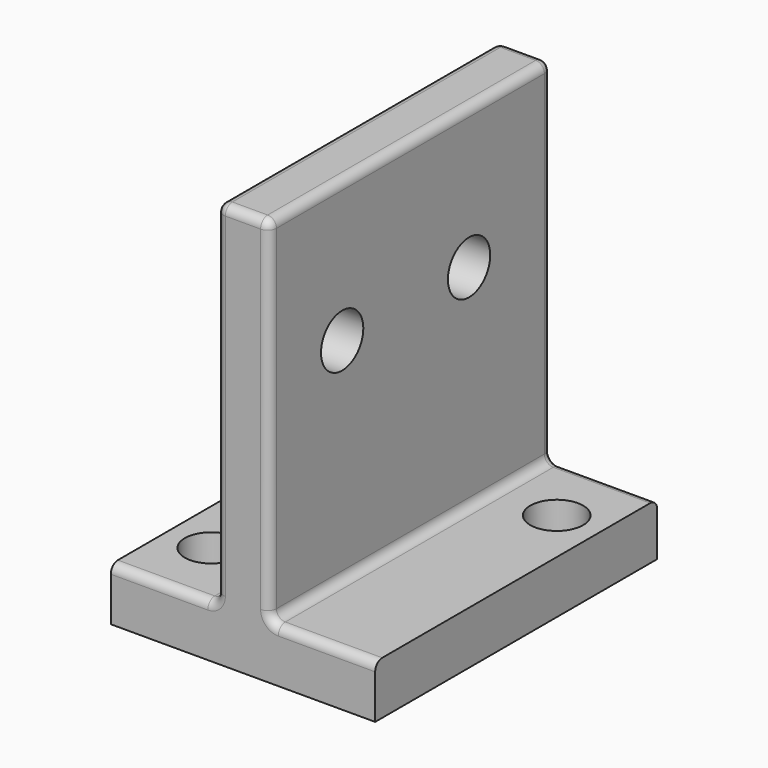
from build123d import *

# Parameters (mm, degrees)
F0_W     = 3
F0_H     = 20
F1_DEPTH = 20
F2_R     = 1.5
F3_DEPTH = 9.001
F4_R     = 1.5
F5_DEPTH = 3.001
F6_R     = 1.5
F7_DEPTH = 25
F8_F1_R  = 0.5
F8_F2_R  = 0.5


with BuildPart() as f1:
    # F0 (on Front) → F1 (new body)
    with BuildSketch(Plane.XZ):
        Rectangle(F0_W, F0_H)
        Polygon((7.5, -10), (1.5, -10), (-1.5, -10), (-7.5, -10), (-7.5, -13), (7.5, -13), align=None)
    extrude(amount=F1_DEPTH)

    # F2 (on face) → F3 (cut, through all)
    with BuildSketch(Plane.YZ.offset(1.5)):
        with Locations((-14.8428049088, 2)):
            Circle(F2_R)
        with Locations((-5.8428049088, 2)):
            Circle(F2_R)
    extrude(amount=-F3_DEPTH, mode=Mode.SUBTRACT)

    # F4 (on face) → F5 (cut, through all)
    with BuildSketch(Plane.XY.offset(-10)):
        with Locations((5, -4)):
            Circle(F4_R)
    extrude(amount=-F5_DEPTH, mode=Mode.SUBTRACT)

    # F6 (on face) → F7 (cut)
    with BuildSketch(Plane.XY.offset(-10)):
        with Locations((-5, -16)):
            Circle(F6_R)
    extrude(amount=-F7_DEPTH, mode=Mode.SUBTRACT)

    # F8: fillet of radius 0.5 on 10 edges, made by hand

    # F8_f1
    f8_f1_edges = [f1.edges().sort_by_distance(p)[0] for p in [
        (1.5, -10, -10),
        (-1.5, -10, -10),
    ]]
    fillet(f8_f1_edges, radius=F8_F1_R)

    # F8_f2
    f8_f2_edges = [f1.edges().sort_by_distance(p)[0] for p in [
        (-1.5, -10, 10),
        (1.5, -20, 0.25),
        (-1.5, -20, 0.25),
        (1.5, -10, 10),
        (-1.5, 0, 0.25),
        (1.5, 0, 0.25),
        (0, -20, 10),
        (0, 0, 10),
        (1.6464466094, 0, -9.8535533906),
        (-1.6464466094, 0, -9.8535533906),
        (-1.6464466094, -20, -9.8535533906),
        (1.6464466094, -20, -9.8535533906),
    ]]
    fillet(f8_f2_edges, radius=F8_F2_R)


solid = f1.part
